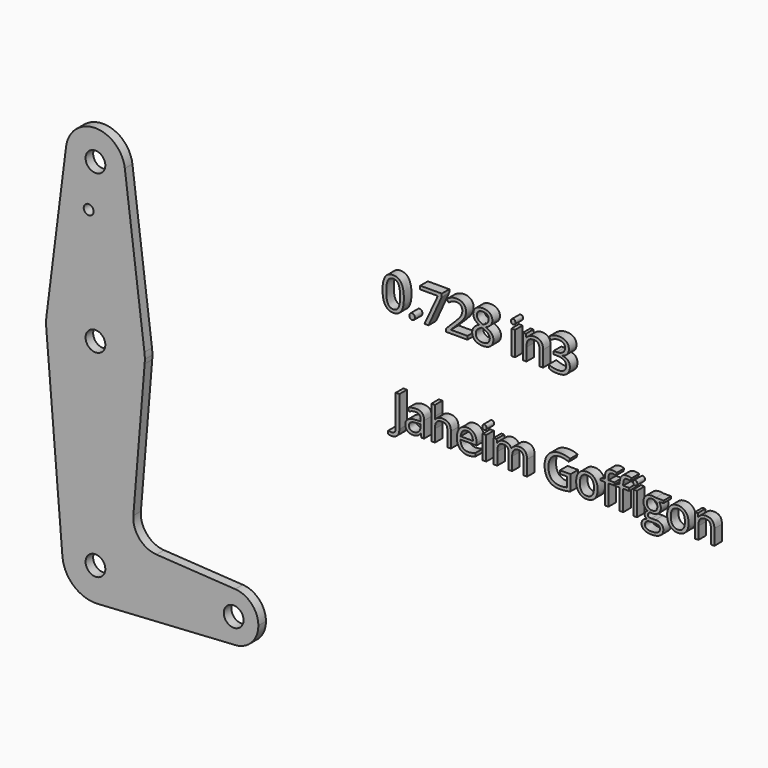
from build123d import *

# Parameters (mm, degrees)
F0_R           = 3.175
F0_R_2         = 1.5875
F0_TEXT_SIZE   = 14.5418724666
F0_TEXT_SIZE_2 = 14.0430936072
F1_DEPTH       = 3.048


# Not quite as in the source:
# - Text() gives the source's letters only with a copy of the font that has no kerning and outlines rounded to 1/6400 em; it was checked with that copy


with BuildPart() as f1:
    # F0 (on Front) → F1 (new body)
    with BuildSketch(Plane.XZ):
        with BuildLine():
            ThreePointArc((-169.6387418761, 54.8803207068), (-160.7849321539, 44.1833908126), (-150.6634489119, 53.6896957068))
            ThreePointArc((-150.6634489119, 53.6896957068), (-150.6821440177, 54.2861789488), (-150.7381559477, 54.8803207068))
            ThreePointArc((-150.7381559477, 54.8803207068), (-160.1884489119, 63.2146957068), (-169.6387418761, 54.8803207068))
        make_face()
        with Locations((-160.1884489119, 53.6896957068)):
            Circle(F0_R, mode=Mode.SUBTRACT)
        with BuildLine():
            ThreePointArc((-150.7381559477, 54.8803207068), (-150.6821440177, 54.2861789488), (-150.6634489119, 53.6896957068))
            ThreePointArc((-150.6634489119, 53.6896957068), (-160.7849321539, 44.1833908126), (-169.6387418761, 54.8803207068))
            Line((-169.6387418761, 54.8803207068), (-175.9389371856, 4.8740707068))
            ThreePointArc((-175.9389371856, 4.8740707068), (-160.1884489119, 18.7646957068), (-144.4379606382, 4.8740707068))
            Line((-144.4379606382, 4.8740707068), (-150.7381559477, 54.8803207068))
        make_face()
        with Locations((-162.370890379, 39.4148957068)):
            Circle(F0_R_2, mode=Mode.SUBTRACT)
        with BuildLine():
            ThreePointArc((-144.3134489119, 2.8896957068), (-144.3446074215, 3.8838344434), (-144.4379606382, 4.8740707068))
            ThreePointArc((-144.4379606382, 4.8740707068), (-160.1884489119, 18.7646957068), (-175.9389371856, 4.8740707068))
            ThreePointArc((-175.9389371856, 4.8740707068), (-176.0597703027, 3.2314299767), (-176.0097536197, 1.5851105842))
            ThreePointArc((-176.0097536197, 1.5851105842), (-160.1884489119, -12.9853042932), (-144.3671442041, 1.5851105842))
            ThreePointArc((-144.3671442041, 1.5851105842), (-144.3268784153, 2.2368508695), (-144.3134489119, 2.8896957068))
        make_face()
        with Locations((-160.1884489119, 2.8896957068)):
            Circle(F0_R, mode=Mode.SUBTRACT)
        with BuildLine():
            ThreePointArc((-144.3671442041, 1.5851105842), (-160.1884489119, -12.9853042932), (-176.0097536197, 1.5851105842))
            Line((-176.0097536197, 1.5851105842), (-170.8090635432, -61.4860535501))
            ThreePointArc((-170.8090635432, -61.4860535501), (-160.6266942753, -49.9626598162), (-149.5317894022, -60.6103042932))
            ThreePointArc((-149.5317894022, -60.6103042932), (-152.4259906453, -67.9115804533), (-159.5365443664, -71.2470054909))
            Line((-159.5365443664, -71.2470054909), (-115.2528847138, -68.5329385558))
            ThreePointArc((-115.2528847138, -68.5329385558), (-123.6759489119, -60.6103042932), (-115.2528847138, -52.6876700306))
            Line((-115.2528847138, -52.6876700306), (-140.5692344954, -51.136075867))
            ThreePointArc((-140.5692344954, -51.136075867), (-146.0930321983, -48.4049859459), (-148.0062027922, -42.5474291601))
            Line((-148.0062027922, -42.5474291601), (-144.3671442041, 1.5851105842))
        make_face()
        with BuildLine():
            ThreePointArc((-149.5317894022, -60.6103042932), (-160.6266942753, -49.9626598162), (-170.8090635432, -61.4860535501))
            ThreePointArc((-170.8090635432, -61.4860535501), (-167.1643245481, -68.666454181), (-159.5365443664, -71.2470054909))
            ThreePointArc((-159.5365443664, -71.2470054909), (-152.4259906453, -67.9115804533), (-149.5317894022, -60.6103042932))
        make_face()
        with Locations((-160.1884489119, -60.6103042932)):
            Circle(F0_R, mode=Mode.SUBTRACT)
        with BuildLine():
            ThreePointArc((-115.2528847138, -52.6876700306), (-123.6759489119, -60.6103042932), (-115.2528847138, -68.5329385558))
            ThreePointArc((-115.2528847138, -68.5329385558), (-109.9566640632, -66.048582533), (-107.8009489119, -60.6103042932))
            ThreePointArc((-107.8009489119, -60.6103042932), (-109.9566640632, -55.1720260534), (-115.2528847138, -52.6876700306))
        make_face()
        with Locations((-115.7384489119, -60.6103042932)):
            Circle(F0_R, mode=Mode.SUBTRACT)
        with Locations((-68.592518568, 42.1903207898)):
            Text('0.728 in3', F0_TEXT_SIZE, font='Open Sans', text_align=(TextAlign.LEFT, TextAlign.BOTTOM))
        with Locations((-64.9332553148, 9.6586206928)):
            Text('Jaheim Goffigon', F0_TEXT_SIZE_2, font='Open Sans', text_align=(TextAlign.LEFT, TextAlign.BOTTOM))
    extrude(amount=F1_DEPTH)


solid = f1.part
